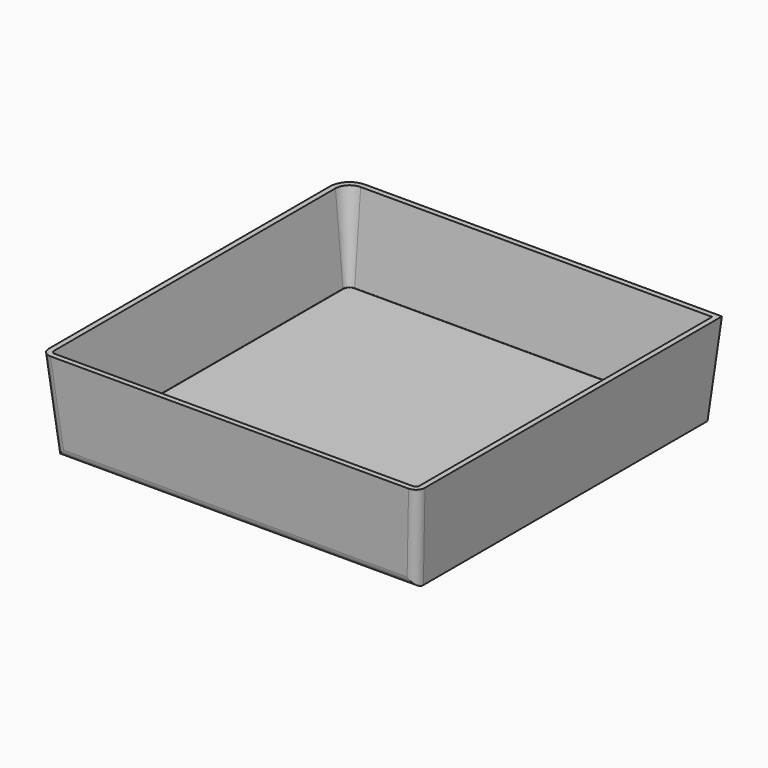
from build123d import *

# Parameters (mm, degrees)
F2_DEPTH               = 50.8
DRAFT_F2_DRAFTED_ANGLE = -5
F3_R                   = 5.08
F4_T                   = -3
F5_R                   = 0.2


# Not quite as in the source:
# - an extrude with a draft is written as a straight extrude whose walls are then drafted


with BuildPart() as f2:
    # F0 (on Top) → F2 (new body)
    with BuildSketch(Plane.XY):
        with BuildLine():
            Line((105.3817194126, 95.5523256148), (-88.2682805874, 95.5523256148))
            ThreePointArc((-88.2682805874, 95.5523256148), (-92.7584086479, 93.6924536754), (-94.6182805874, 89.2023256148))
            Line((-94.6182805874, 89.2023256148), (-94.6182805874, -106.6376079099))
            Line((-94.6182805874, -106.6376079099), (105.3817194126, -106.6376079099))
            Line((105.3817194126, -106.6376079099), (105.3817194126, 95.5523256148))
        make_face()
    extrude(amount=F2_DEPTH)

    # draft_F2_drafted
    draft_f2_drafted_walls = [f2.faces().sort_by_distance(p)[0] for p in [
        (105.3817194126, -5.5426411475, 33.8666666667),
        (8.5567194126, 95.5523256148, 33.8666666667),
        (-92.7584086479, 93.6924536754, 33.8666666667),
        (-94.6182805874, -8.7176411475, 33.8666666667),
        (5.3817194126, -106.6376079099, 33.8666666667),
    ]]
    draft(draft_f2_drafted_walls, neutral_plane=Plane.XY, angle=DRAFT_F2_DRAFTED_ANGLE)

    # F3
    f3_edges = [f2.edges().sort_by_distance(p)[0] for p in [
        (5.381719, -106.637608, 0),
        (107.603931, -108.85982, 25.4),
        (-96.840493, -108.85982, 25.4),
    ]]
    fillet(f3_edges, radius=F3_R)

    # F4
    f4_openings = [f2.faces().sort_by_distance(p)[0] for p in [
        (5.439631, -5.575189, 50.8),
    ]]
    offset(amount=F4_T, openings=f4_openings)

    # F5
    f5_edges = [f2.edges().sort_by_distance(p)[0] for p in [
        (7.182223, 92.803332, 3),
        (5.381719, -101.982646, 3),
        (102.63107, -101.899653, 3),
        (102.632726, -4.506599, 3),
        (-90.814577, 91.748622, 3),
        (-91.869287, -6.307102, 3),
        (-91.867631, -101.899653, 3),
        (102.014838, -103.387873, 3.546463),
        (-91.251399, -103.387873, 3.546463),
    ]]
    fillet(f5_edges, radius=F5_R)


solid = f2.part
